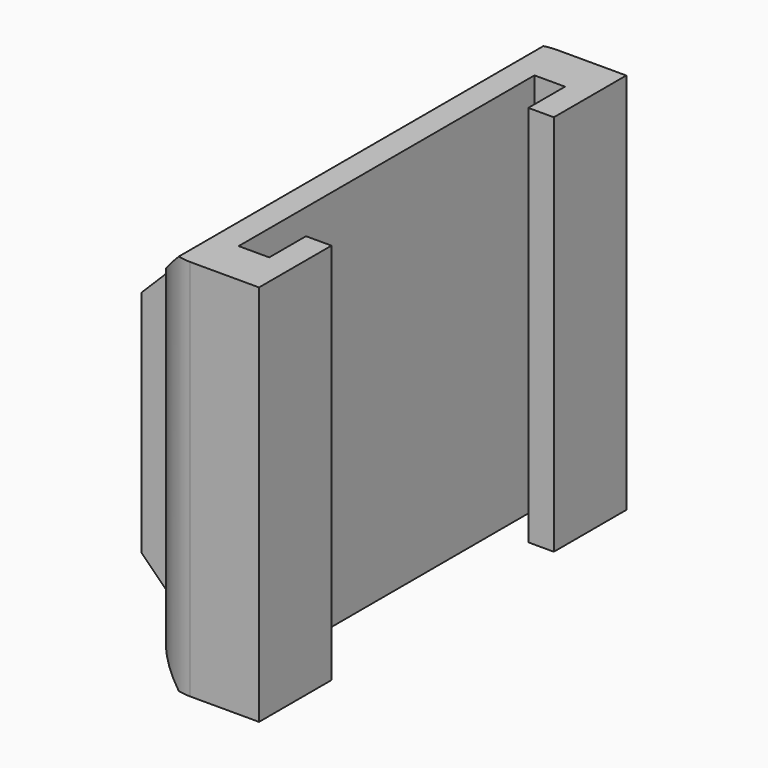
from build123d import *

# Parameters (mm, degrees)
F1_DEPTH = 15
F2_R     = 1.99999
F3_SIZE  = 3


# Not quite as in the source:
# - a fillet or chamfer is up to 0.001 mm smaller than in the source, because OpenCascade refuses the exact size


with BuildPart() as f1:
    # F0 (on Top) → F1 (new body)
    with BuildSketch(Plane.XY):
        Polygon((0, 16), (0, 2), (1.5, 2), (1.5, 0), (6.2, 0), (6.2, 3.55), (5.2, 3.55), (5.2, 1.75), (4, 1.75), (4, 16.25), (5.2, 16.25), (5.2, 14.45), (6.2, 14.45), (6.2, 18), (1.5, 18), (1.5, 16), align=None)
    extrude(amount=F1_DEPTH)

    # F2 (radius 2 in the source; OpenCascade refuses exactly that, so slightly less here)
    f2_edges = [f1.edges().sort_by_distance(p)[0] for p in [
        (1.5, 0, 7.5),
        (1.5, 18, 7.5),
    ]]
    fillet(f2_edges, radius=F2_R)

    # F3
    f3_edges = [f1.edges().sort_by_distance(p)[0] for p in [
        (0, 9, 0),
        (0, 9, 15),
    ]]
    chamfer(f3_edges, length=F3_SIZE)


solid = f1.part
